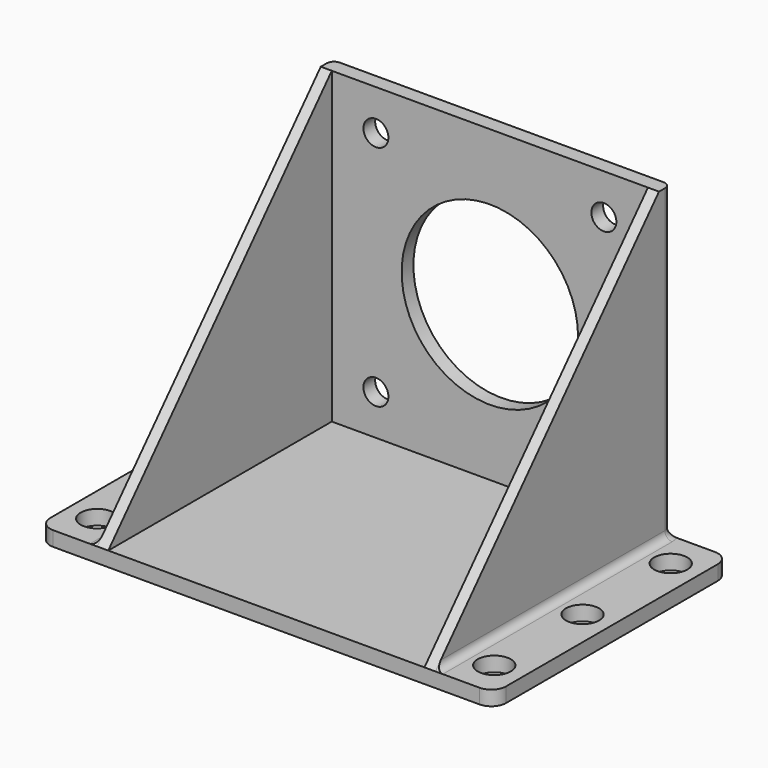
from build123d import *

# Parameters (mm, degrees)
F0_W         = 62
F0_H         = 40
F0_R         = 2.25
F1_DEPTH     = 2
F2_W         = 46
F2_H         = 42
F2_R         = 1.7
F2_R_2       = 12
F3_DEPTH     = 2
F5_DEPTH     = 1.5
F6_R         = 2
F7_R         = 1
F8_T4_DEPTH  = 41.5
F8_T9_ANGLE  = 233.2969892374
F8_T15_ANGLE = 233.2969892374
F8_T21_DEPTH = 41.5


# Not quite as in the source:
# - a fillet or chamfer that OpenCascade refuses, or shapes differently, is made with other operations: its cross-section is extruded or revolved along the edge and cut away or added
# - a pattern or mirror of a feature is missing from the dataset's text; its kind, count and spacing are read off the source's solid


with BuildPart() as f1:
    # F0 (on Top) → F1 (new body)
    with BuildSketch(Plane.XY):
        with Locations((0, -20)):
            Rectangle(F0_W, F0_H)
        with Locations((-27, -35)):
            Circle(F0_R, mode=Mode.SUBTRACT)
        with Locations((27, -35)):
            Circle(F0_R, mode=Mode.SUBTRACT)
        with Locations((-27, -20)):
            Circle(F0_R, mode=Mode.SUBTRACT)
        with Locations((-27, -5)):
            Circle(F0_R, mode=Mode.SUBTRACT)
        with Locations((27, -20)):
            Circle(F0_R, mode=Mode.SUBTRACT)
        with Locations((27, -5)):
            Circle(F0_R, mode=Mode.SUBTRACT)
    extrude(amount=F1_DEPTH)

    # F2 (on Front) → F3 (join)
    with BuildSketch(Plane.XZ):
        with Locations((0, 23)):
            Rectangle(F2_W, F2_H)
        with Locations((-15.5, 7.5)):
            Circle(F2_R, mode=Mode.SUBTRACT)
        with Locations((15.5, 7.5)):
            Circle(F2_R, mode=Mode.SUBTRACT)
        with Locations((-15.5, 38.5)):
            Circle(F2_R, mode=Mode.SUBTRACT)
        with Locations((0, 23)):
            Circle(F2_R_2, mode=Mode.SUBTRACT)
        with Locations((15.5, 38.5)):
            Circle(F2_R, mode=Mode.SUBTRACT)
    extrude(amount=F3_DEPTH)

    # F4 (on face) → F5 (join)
    with BuildSketch(Plane.YZ.offset(23)):
        Polygon((-2, 2), (-2, 44), (-40, 2), align=None)
    f5 = extrude(amount=-F5_DEPTH)

    # F5_copies: F5 across plane
    add(f5.mirror(Plane(origin=(0, 0, 0), x_dir=(0, 0, -1), z_dir=(-1, 0, 0))))

    # F6
    f6_edges = [f1.edges().sort_by_distance(p)[0] for p in [
        (31, -40, 1),
        (31, 0, 1),
        (-31, 0, 1),
        (-31, -40, 1),
    ]]
    fillet(f6_edges, radius=F6_R)

    # F7
    f7_edges = [f1.edges().sort_by_distance(p)[0] for p in [
        (-23, 0, 23),
        (23, 0, 23),
    ]]
    fillet(f7_edges, radius=F7_R)

    # F8: fillet of radius 1 on 4 edges, made by hand


with BuildPart() as f8_tool2:
    # F8_s3 → F8_t4 (new body)
    with BuildSketch(Plane.XZ.offset(1)):
        with BuildLine():
            ThreePointArc((24, 2), (23.2928932188, 2.2928932188), (23, 3))
            Line((23, 3), (23, 2))
            Line((23, 2), (24, 2))
        make_face()
    extrude(amount=F8_T4_DEPTH)

    split(bisect_by=Plane(origin=(0, -22.9900249377, 20.8004987531), x_dir=(1, 0, 0), z_dir=(0, 0.7415357791, -0.670913324)), keep=Keep.TOP)


with BuildPart() as f1_1:
    add(f1.part)

    # F8_t1: union F8_tool2
    add(f8_tool2.part)


with BuildPart() as f8_tool7:
    # F8_s8 → F8_t9 (revolve)
    with BuildSketch(Plane(origin=(14.6206404523, -10.8990847056, 0), x_dir=(0, 0, 1), z_dir=(0.8017442393, -0.5976672776, 0))):
        with BuildLine():
            ThreePointArc((3, -11.3469358686), (2.2928932188, -11.0540426498), (2, -10.3469358686))
            Line((2, -10.3469358686), (2, -11.3469358686))
            Line((2, -11.3469358686), (3, -11.3469358686))
        make_face()
    revolve(axis=Axis((22, -1, 2), (0, 0, -1)), revolution_arc=F8_T9_ANGLE)

    split(bisect_by=Plane.XZ, keep=Keep.TOP)

    split(bisect_by=Plane.XZ.offset(2), keep=Keep.BOTTOM)


with BuildPart() as f1_2:
    add(f1_1.part)

    # F8_t6: union F8_tool7
    add(f8_tool7.part)


with BuildPart() as f8_tool13:
    # F8_s14 → F8_t15 (revolve)
    with BuildSketch(Plane(origin=(-14.6206404523, -10.8990847056, 0), x_dir=(0, 0, 1), z_dir=(-0.8017442393, -0.5976672776, 0))):
        with BuildLine():
            ThreePointArc((3, 11.3469358686), (2.2928932188, 11.0540426498), (2, 10.3469358686))
            Line((2, 10.3469358686), (2, 11.3469358686))
            Line((2, 11.3469358686), (3, 11.3469358686))
        make_face()
    revolve(axis=Axis((-22, -1, 2), (0, 0, 1)), revolution_arc=F8_T15_ANGLE)

    split(bisect_by=Plane.XZ, keep=Keep.TOP)

    split(bisect_by=Plane.XZ.offset(2), keep=Keep.BOTTOM)


with BuildPart() as f1_3:
    add(f1_2.part)

    # F8_t12: union F8_tool13
    add(f8_tool13.part)


with BuildPart() as f8_tool19:
    # F8_s20 → F8_t21 (new body)
    with BuildSketch(Plane.XZ.offset(1)):
        with BuildLine():
            ThreePointArc((-24, 2), (-23.2928932188, 2.2928932188), (-23, 3))
            Line((-23, 3), (-23, 2))
            Line((-23, 2), (-24, 2))
        make_face()
    extrude(amount=F8_T21_DEPTH)

    split(bisect_by=Plane(origin=(0, -22.9900249377, 20.8004987531), x_dir=(1, 0, 0), z_dir=(0, 0.7415357791, -0.670913324)), keep=Keep.TOP)


with BuildPart() as f1_4:
    add(f1_3.part)

    # F8_t18: union F8_tool19
    add(f8_tool19.part)


solid = f1_4.part
